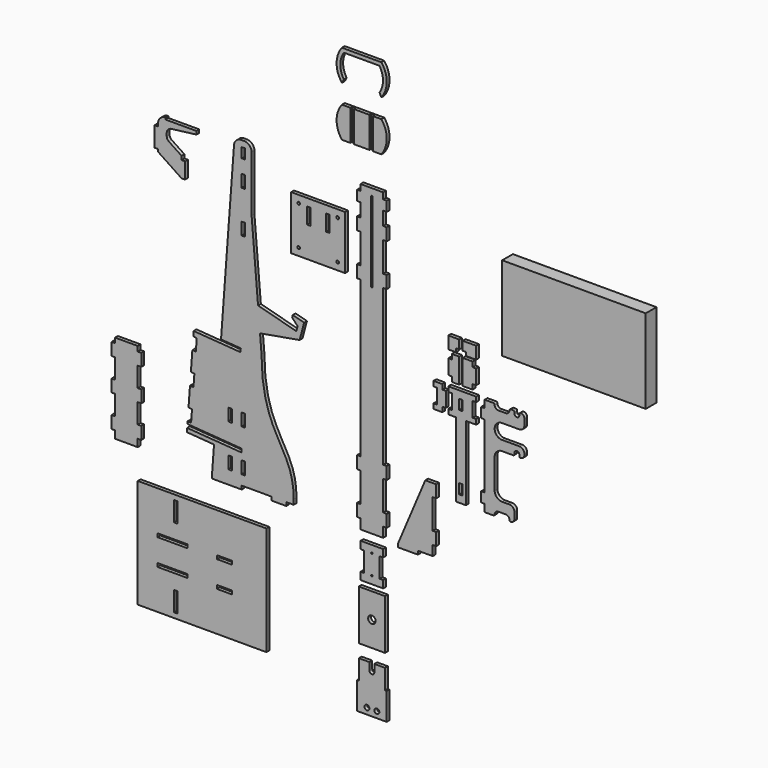
from build123d import *

# Parameters (mm, degrees)
F1_W     = 18.034
F1_H     = 63.5
F1_W_2   = 101.6
F1_H_2   = 18.034
F2_DEPTH = 18.034
F1_H_3   = 50.8
F1_W_3   = 152.4
F1_W_4   = 76.2
F1_W_5   = 276.2
F1_H_4   = 276.2
F1_R     = 6.985
F1_H_5   = 82.55
F1_R_2   = 12.7
F1_W_6   = 8.8265
F1_H_6   = 139.7
F1_W_7   = 9.2075
F1_H_7   = 101.6
F1_W_8   = 79.883
F1_H_8   = 158.75
F1_R_3   = 3.81
F1_W_9   = 134.366
F1_H_9   = 256.286
F1_R_4   = 19.05
F3_DEPTH = 9.017
F1_W_10  = 736.6
F1_H_10  = 431.8
F4_DEPTH = 68.58
F6_DEPTH = 18.034
F5_W     = 18.034
F5_H     = 50.8
F5_H_2   = 25.4
F5_H_3   = 76.2


# Not quite as in the source:
# - a variable given as a bare number and used for a length is read in inches; the dataset says mm whatever the document's units were


with BuildPart() as f2:
    # F1 (on Front) → F2 (new body)
    with BuildSketch(Plane.XZ):
        Polygon((312.166, -462.8884474277), (312.166, -399.3884474277), (274.066, -399.3884474277), (134.366, -729.5884474277), (235.966, -729.5884474277), (312.166, -729.5884474277), (312.166, -678.7884474277), (312.166, -615.2884474277), align=None)
        with Locations((321.183, -431.1384474277)):
            Rectangle(F1_W, F1_H)
        with Locations((321.183, -647.0384474277)):
            Rectangle(F1_W, F1_H)
        with Locations((185.166, -738.6054474277)):
            Rectangle(F1_W_2, F1_H_2)
    extrude(amount=F2_DEPTH)


with BuildPart() as f2b:
    # F1 (on Front) → F2, piece 2 (new body)
    with BuildSketch(Plane.XZ):
        with Locations((-1326.515, -329.5384474277)):
            Rectangle(F1_W, F1_H)
        with Locations((-1326.515, -494.6384474277)):
            Rectangle(F1_W, F1_H)
        with Locations((-1192.149, -494.6384474277)):
            Rectangle(F1_W, F1_H)
        with Locations((-1192.149, -329.5384474277)):
            Rectangle(F1_W, F1_H)
        Polygon((-1317.498, -729.5884474277), (-1201.166, -729.5884474277), (-1201.166, -691.4884474277), (-1201.166, -627.9884474277), (-1201.166, -526.3884474277), (-1201.166, -462.8884474277), (-1201.166, -361.2884474277), (-1201.166, -297.7884474277), (-1201.166, -272.3884474277), (-1317.498, -272.3884474277), (-1317.498, -297.7884474277), (-1317.498, -361.2884474277), (-1317.498, -462.8884474277), (-1317.498, -526.3884474277), (-1317.498, -627.9884474277), (-1317.498, -691.4884474277), align=None)
        with Locations((-1326.515, -659.7384474277)):
            Rectangle(F1_W, F1_H)
        with Locations((-1192.149, -659.7384474277)):
            Rectangle(F1_W, F1_H)
    extrude(amount=F2_DEPTH)


with BuildPart() as f2c:
    # F1 (on Front) → F2, piece 3 (new body)
    with BuildSketch(Plane.XZ):
        with BuildLine():
            Line((-707.3307957356, 795.6225112467), (-712.216, 729.5884474277))
            Line((-712.216, 729.5884474277), (-773.8601407698, -103.6649653974))
            Line((-773.8601407698, -103.6649653974), (-672.5370356253, -111.1608551959))
            Line((-672.5370356253, -111.1608551959), (-673.8675560645, -129.1457063591))
            Line((-673.8675560645, -129.1457063591), (-775.190661209, -121.6498165606))
            Line((-775.190661209, -121.6498165606), (-807.0481928526, -552.2730134248))
            Line((-807.0481928526, -552.2730134248), (-667.766, -562.5771189596))
            Line((-667.766, -562.5771189596), (-667.766, -580.6604021099))
            Line((-667.766, -580.6604021099), (-808.3787132919, -570.257864588))
            Line((-808.3787132919, -570.257864588), (-809.8591515271, -590.269177854))
            Line((-809.8591515271, -590.269177854), (-820.166, -729.5884474277))
            Line((-820.166, -729.5884474277), (-667.766, -729.5884474277))
            Line((-667.766, -729.5884474277), (-515.366, -729.5884474277))
            Line((-515.366, -729.5884474277), (-439.166, -729.5884474277))
            Line((-439.166, -729.5884474277), (-401.066, -729.5884474277))
            Line((-401.066, -729.5884474277), (-401.066, -704.1884474277))
            add(Edge.make_bspline(
                [(-566.166, -102.5384474277), (-566.166, -468.3954715729), (-401.066, -468.3954715729), (-401.066, -704.1884474277)],
                knots=[0, 0, 0, 0, 623.8916031652, 623.8916031652, 623.8916031652, 623.8916031652], degree=3))
            Line((-566.166, -102.5384474277), (-573.766897729, -11.3276746799))
            Line((-573.766897729, -11.3276746799), (-583.9832928314, 111.2690665494))
            Line((-583.9832928314, 111.2690665494), (-616.966, 507.0615525723))
            Line((-616.966, 507.0615525723), (-616.966, 544.2178131268))
            Line((-616.966, 544.2178131268), (-616.966, 627.7115525723))
            Line((-616.966, 627.7115525723), (-616.966, 659.4615525723))
            Line((-616.966, 659.4615525723), (-616.966, 761.0615525723))
            Line((-616.966, 761.0615525723), (-616.966, 792.8115525723))
            ThreePointArc((-616.966, 792.8115525723), (-628.1252316368, 819.7523209355), (-655.066, 830.9115525723))
            Line((-655.066, 830.9115525723), (-669.3346313064, 830.9115525723))
            ThreePointArc((-669.3346313064, 830.9115525723), (-695.2625359123, 820.7284607597), (-707.3307957356, 795.6225112467))
        make_face()
        with Locations((-727.583, -647.0384474277)):
            Rectangle(F1_W, F1_H, mode=Mode.SUBTRACT)
        with Locations((-658.749, -647.0384474277)):
            Rectangle(F1_W, F1_H, mode=Mode.SUBTRACT)
        with Locations((-727.583, -431.1384474277)):
            Rectangle(F1_W, F1_H, mode=Mode.SUBTRACT)
        with Locations((-658.749, -431.1384474277)):
            Rectangle(F1_W, F1_H, mode=Mode.SUBTRACT)
        with Locations((-658.749, 431.1384474277)):
            Rectangle(F1_W, F1_H, mode=Mode.SUBTRACT)
        with Locations((-658.749, 647.0384474277)):
            Rectangle(F1_W, F1_H, mode=Mode.SUBTRACT)
        with Locations((-658.749, 773.7615525723)):
            Rectangle(F1_W, F1_H_3, mode=Mode.SUBTRACT)
        Polygon((-387.7071649295, 58.6770365845), (-583.9832928314, 111.2690665494), (-573.766897729, -11.3276746799), (-370.5684031555, 24.5017023527), (-347.5593900459, 110.3725083098), (-405.8288655168, 125.9857672056), (-409.1158673896, 113.7185092117), (-381.1331611839, 83.2115525723), align=None)
        Polygon((-807.0481928526, -552.2730134248), (-775.190661209, -121.6498165606), (-914.5099307827, -111.3429680876), (-916.3839032324, -136.6737443738), (-898.3990520692, -138.004264813), (-903.0839831933, -201.3312055283), (-921.0688343564, -200.0006850891), (-928.5647241549, -301.3237902336), (-910.5798729918, -302.6543106729), (-915.2648041158, -365.9812513882), (-933.249655279, -364.650730949), (-940.7455450775, -465.9738360935), (-922.7606939143, -467.3043565327), (-927.4456250384, -530.631297248), (-945.4304762015, -529.3007768088), (-946.3674624264, -541.9661649519), align=None)
        Polygon((-809.8591515271, -590.269177854), (-808.3787132919, -570.257864588), (-947.6979828656, -559.951016115), (-949.1784211008, -579.9623293811), align=None)
        with Locations((-743.966, -738.6054474277)):
            Rectangle(F1_W_3, F1_H_2)
        with Locations((-477.266, -738.6054474277)):
            Rectangle(F1_W_4, F1_H_2)
    extrude(amount=F2_DEPTH)


with BuildPart() as f2d:
    # F1 (on Front) → F2, piece 4 (new body)
    with BuildSketch(Plane.XZ):
        with Locations((67.183, 647.0384474277)):
            Rectangle(F1_W, F1_H)
        with Locations((67.183, 431.1384474277)):
            Rectangle(F1_W, F1_H)
        with Locations((-67.183, 431.1384474277)):
            Rectangle(F1_W, F1_H)
        with Locations((-67.183, 647.0384474277)):
            Rectangle(F1_W, F1_H)
        with Locations((-67.183, -431.1384474277)):
            Rectangle(F1_W, F1_H)
        with Locations((-67.183, -647.0384474277)):
            Rectangle(F1_W, F1_H)
        with Locations((67.183, -647.0384474277)):
            Rectangle(F1_W, F1_H)
        with Locations((67.183, -431.1384474277)):
            Rectangle(F1_W, F1_H)
        Polygon((-58.166, -678.7884474277), (-58.166, -729.5884474277), (58.166, -729.5884474277), (58.166, -678.7884474277), (58.166, -615.2884474277), (58.166, -462.8884474277), (58.166, -399.3884474277), (58.166, 399.3884474277), (58.166, 462.8884474277), (58.166, 615.2884474277), (58.166, 678.7884474277), (58.166, 729.5884474277), (58.166, 748.3615525723), (58.166, 799.1615525723), (58.166, 830.9115525723), (-58.166, 830.9115525723), (-58.166, 799.1615525723), (-58.166, 748.3615525723), (-58.166, 729.5884474277), (-58.166, 678.7884474277), (-58.166, 615.2884474277), (-58.166, 462.8884474277), (-58.166, 399.3884474277), (-58.166, -399.3884474277), (-58.166, -462.8884474277), (-58.166, -615.2884474277), align=None)
        with BuildLine():
            Line((-3.81, 386.4115525723), (-3.81, 792.8115525723))
            ThreePointArc((-3.81, 792.8115525723), (0, 796.6215525723), (3.81, 792.8115525723))
            Line((3.81, 792.8115525723), (3.81, 386.4115525723))
            ThreePointArc((3.81, 386.4115525723), (0, 382.6015525723), (-3.81, 386.4115525723))
        make_face(mode=Mode.SUBTRACT)
        with Locations((-67.183, 773.7615525723)):
            Rectangle(F1_W, F1_H_3)
        with Locations((67.183, 773.7615525723)):
            Rectangle(F1_W, F1_H_3)
    extrude(amount=F2_DEPTH)


with BuildPart() as f2e:
    # F1 (on Front) → F2, piece 5 (new body)
    with BuildSketch(Plane.XZ):
        with Locations((-275.666, 540.4115525723)):
            Rectangle(F1_W_5, F1_H_4)
        with Locations((-375.666, 440.4115525723)):
            Circle(F1_R, mode=Mode.SUBTRACT)
        with Locations((-324.6245, 599.1365525723)):
            Rectangle(F1_W, F1_H_5, mode=Mode.SUBTRACT)
        with Locations((-375.666, 640.4115525723)):
            Circle(F1_R, mode=Mode.SUBTRACT)
        with Locations((-175.666, 440.4115525723)):
            Circle(F1_R, mode=Mode.SUBTRACT)
        with Locations((-226.7075, 599.1365525723)):
            Rectangle(F1_W, F1_H_5, mode=Mode.SUBTRACT)
        with Locations((-175.666, 640.4115525723)):
            Circle(F1_R, mode=Mode.SUBTRACT)
    extrude(amount=F2_DEPTH)


with BuildPart() as f2f:
    # F1 (on Front) → F2, piece 6 (new body)
    with BuildSketch(Plane.XZ):
        with BuildLine():
            ThreePointArc((-143.8170263099, 1275.6884474277), (-161.925, 1336.0134474277), (-143.8170263099, 1396.3384474277))
            Line((-143.8170263099, 1396.3384474277), (39.0420263099, 1396.3384474277))
            ThreePointArc((39.0420263099, 1396.3384474277), (57.15, 1336.0134474277), (39.0420263099, 1275.6884474277))
            Line((39.0420263099, 1275.6884474277), (48.7774866864, 1256.6384474277))
            ThreePointArc((48.7774866864, 1256.6384474277), (76.2, 1336.0134474277), (48.7774866864, 1415.3884474277))
            Line((48.7774866864, 1415.3884474277), (-153.5524866864, 1415.3884474277))
            ThreePointArc((-153.5524866864, 1415.3884474277), (-180.975, 1336.0134474277), (-153.5524866864, 1256.6384474277))
            Line((-153.5524866864, 1256.6384474277), (-143.8170263099, 1275.6884474277))
        make_face()
    extrude(amount=F2_DEPTH)


with BuildPart() as f2g:
    # F1 (on Front) → F2, piece 7 (new body)
    with BuildSketch(Plane.XZ):
        with BuildLine():
            Line((-12.5095, -1313.7884474277), (-66.9925, -1313.7884474277))
            Line((-66.9925, -1313.7884474277), (-66.9925, -1415.3884474277))
            Line((-66.9925, -1415.3884474277), (-66.9925, -1555.0884474277))
            Line((-66.9925, -1555.0884474277), (67.3735, -1555.0884474277))
            Line((67.3735, -1555.0884474277), (67.3735, -1415.3884474277))
            Line((67.3735, -1415.3884474277), (67.3735, -1313.7884474277))
            Line((67.3735, -1313.7884474277), (12.8905, -1313.7884474277))
            Line((12.8905, -1313.7884474277), (12.8905, -1351.8884474277))
            ThreePointArc((12.8905, -1351.8884474277), (0.1905, -1364.5884474277), (-12.5095, -1351.8884474277))
            Line((-12.5095, -1351.8884474277), (-12.5095, -1313.7884474277))
        make_face()
        with Locations((-25.2095, -1523.3384474277)):
            Circle(F1_R_2, mode=Mode.SUBTRACT)
        with Locations((25.5905, -1523.3384474277)):
            Circle(F1_R_2, mode=Mode.SUBTRACT)
        with Locations((71.78675, -1485.2384474277)):
            Rectangle(F1_W_6, F1_H_6)
        with Locations((-71.59625, -1485.2384474277)):
            Rectangle(F1_W_7, F1_H_6)
    extrude(amount=F2_DEPTH)


with BuildPart() as f2h:
    # F1 (on Front) → F2, piece 8 (new body)
    with BuildSketch(Plane.XZ):
        with BuildLine():
            Line((-976.2594103813, 640.4115525723), (-976.2594103813, 659.4615525723))
            Line((-976.2594103813, 659.4615525723), (-1041.1487953654, 702.7211425617))
            ThreePointArc((-1041.1487953654, 702.7211425617), (-1049.45394519, 711.8700287293), (-1052.4594103813, 723.8552200379))
            Line((-1052.4594103813, 723.8552200379), (-1052.4594103813, 738.6388842214))
            ThreePointArc((-1052.4594103813, 738.6388842214), (-1046.101236047, 755.4486693276), (-1030.2098926399, 763.8427422899))
            Line((-1030.2098926399, 763.8427422899), (-900.0594103813, 780.1115525723))
            Line((-900.0594103813, 780.1115525723), (-900.0594103813, 796.4945525723))
            Line((-900.0594103813, 796.4945525723), (-1058.8094103813, 796.4945525723))
            Line((-1058.8094103813, 796.4945525723), (-1058.8094103813, 805.5115525723))
            ThreePointArc((-1058.8094103813, 805.5115525723), (-1085.7501787445, 794.3523209355), (-1096.9094103813, 767.4115525723))
            Line((-1096.9094103813, 767.4115525723), (-1096.9094103813, 752.5948859056))
            Line((-1096.9094103813, 752.5948859056), (-1096.9094103813, 650.9948859056))
            Line((-1096.9094103813, 650.9948859056), (-1096.9094103813, 638.2948859056))
            Line((-1096.9094103813, 638.2948859056), (-976.2594103813, 557.8615525723))
            Line((-976.2594103813, 557.8615525723), (-958.2254103813, 557.8615525723))
            Line((-958.2254103813, 557.8615525723), (-958.2254103813, 640.4115525723))
            Line((-958.2254103813, 640.4115525723), (-976.2594103813, 640.4115525723))
        make_face()
        with Locations((-1105.9264103813, 701.7948859056)):
            Rectangle(F1_W, F1_H_7)
    extrude(amount=F2_DEPTH)


with BuildPart() as f2i:
    # F1 (on Front) → F2, piece 9 (new body)
    with BuildSketch(Plane.XZ):
        with BuildLine():
            ThreePointArc((48.7774866864, 999.4634474277), (69.1511726145, 1036.8492081472), (76.2, 1078.8384474277))
            ThreePointArc((76.2, 1078.8384474277), (69.1511726145, 1120.8276867083), (48.7774866864, 1158.2134474277))
            Line((48.7774866864, 1158.2134474277), (5.588, 1158.2134474277))
            Line((5.588, 1158.2134474277), (5.588, 999.4634474277))
            Line((5.588, 999.4634474277), (48.7774866864, 999.4634474277))
        make_face()
    extrude(amount=F2_DEPTH)



with BuildPart() as f2j:
    # F1 (on Front) → F2, piece 10 (new body)
    with BuildSketch(Plane.XZ):
        with Locations((-52.3875, 1078.8384474277)):
            Rectangle(F1_W_8, F1_H_8)
    extrude(amount=F2_DEPTH)


with BuildPart() as f2k:
    # F1 (on Front) → F2, piece 11 (new body)
    with BuildSketch(Plane.XZ):
        with BuildLine():
            ThreePointArc((-153.5524866864, 1158.2134474277), (-173.9261725074, 1120.8276870182), (-180.975, 1078.8384480836))
            ThreePointArc((-180.975, 1078.8384480836), (-173.9261727216, 1036.8492084571), (-153.5524866864, 999.4634474277))
            Line((-153.5524866864, 999.4634474277), (-110.363, 999.4634474277))
            Line((-110.363, 999.4634474277), (-110.363, 1158.2134474277))
            Line((-110.363, 1158.2134474277), (-153.5524866864, 1158.2134474277))
        make_face()
    extrude(amount=F2_DEPTH)


with BuildPart() as f2l:
    # F1 (on Front) → F2, piece 12 (new body)
    with BuildSketch(Plane.XZ):
        Polygon((58.166, -780.3884474277), (-57.785, -780.3884474277), (-57.785, -818.4884474277), (-39.751, -818.4884474277), (-39.751, -920.0884474277), (-57.785, -920.0884474277), (-57.785, -958.1884474277), (58.166, -958.1884474277), (58.166, -920.0884474277), (40.132, -920.0884474277), (40.132, -818.4884474277), (58.166, -818.4884474277), align=None)
        with Locations((0.1905, -920.0884474277)):
            Circle(F1_R_3, mode=Mode.SUBTRACT)
        with Locations((0.1905, -818.4884474277)):
            Circle(F1_R_3, mode=Mode.SUBTRACT)
    extrude(amount=F2_DEPTH)


with BuildPart() as f2m:
    # F1 (on Front) → F2, piece 13 (new body)
    with BuildSketch(Plane.XZ):
        with Locations((0.1905, -1118.0814474277)):
            Rectangle(F1_W_9, F1_H_9)
        with Locations((0, -1118.0814474277)):
            Circle(F1_R_4, mode=Mode.SUBTRACT)
    extrude(amount=F2_DEPTH)


with BuildPart() as f2n:
    # F1 (on Front) → F2, piece 14 (new body)
    with BuildSketch(Plane.XZ):
        Polygon((-540.766, -881.9884474277), (-1201.166, -881.9884474277), (-1201.166, -1440.7884474277), (-540.766, -1440.7884474277), (-540.766, -1161.3884474277), (-540.766, -994.3783283234), align=None)
        with Locations((-1006.983, -1364.5884474277)):
            Rectangle(F1_W, F1_H_7, mode=Mode.SUBTRACT)
        with Locations((-1023.366, -1228.5714474277)):
            Rectangle(F1_W_3, F1_H_2, mode=Mode.SUBTRACT)
        with Locations((-756.666, -1228.5714474277)):
            Rectangle(F1_W_4, F1_H_2, mode=Mode.SUBTRACT)
        with Locations((-1023.366, -1094.2054474277)):
            Rectangle(F1_W_3, F1_H_2, mode=Mode.SUBTRACT)
        with Locations((-1006.983, -958.1884474277)):
            Rectangle(F1_W, F1_H_7, mode=Mode.SUBTRACT)
        with Locations((-756.666, -1094.2054474277)):
            Rectangle(F1_W_4, F1_H_2, mode=Mode.SUBTRACT)
    extrude(amount=F2_DEPTH)


with BuildPart() as f2i_1:
    add(f2i.part)

    add(f2j.part)  # F3 merges F2j

    add(f2k.part)  # F3 merges F2k
    # F1 (on Front) → F3 (join)
    with BuildSketch(Plane.XZ):
        with Locations((-101.346, 1078.8384474277)):
            Rectangle(F1_W, F1_H_8)
        with Locations((-3.429, 1078.8384474277)):
            Rectangle(F1_W, F1_H_8)
    extrude(amount=F3_DEPTH)


with BuildPart() as f4:
    # F1 (on Front) → F4 (new body)
    with BuildSketch(Plane.XZ):
        with Locations((1077.2890025383, 540.4115525723)):
            Rectangle(F1_W_10, F1_H_10)
    extrude(amount=F4_DEPTH)


with BuildPart() as f6:
    # F5 (on Front) → F6 (new body)
    with BuildSketch(Plane.XZ):
        Polygon((410.083, 114.3), (410.083, 88.9), (448.183, 88.9), (448.183, 215.9), (410.083, 215.9), (410.083, 190.5), (392.049, 190.5), (392.049, 114.3), align=None)
    extrude(amount=F6_DEPTH)


with BuildPart() as f6b:
    # F5 (on Front) → F6, piece 2 (new body)
    with BuildSketch(Plane.XZ):
        Polygon((466.217, 215.9), (466.217, 88.9), (517.017, 88.9), (517.017, 114.3), (535.051, 114.3), (535.051, 190.5), (517.017, 190.5), (517.017, 215.9), align=None)
    extrude(amount=F6_DEPTH)


with BuildPart() as f6c:
    # F5 (on Front) → F6, piece 3 (new body)
    with BuildSketch(Plane.XZ):
        Polygon((504.317, 63.5), (410.083, 63.5), (410.083, 38.1), (410.083, -38.1), (410.083, -63.5), (431.8, -63.5), (431.8, -444.5), (482.6, -444.5), (482.6, -63.5), (504.317, -63.5), (517.017, -63.5), (517.017, -38.1), (517.017, 38.1), (517.017, 63.5), align=None)
        with Locations((457.2, -381)):
            Rectangle(F5_W, F5_H, mode=Mode.SUBTRACT)
        with Locations((457.2, 0)):
            Rectangle(F5_W, F5_H, mode=Mode.SUBTRACT)
        with Locations((401.066, 50.8)):
            Rectangle(F5_W, F5_H_2)
        with Locations((401.066, -50.8)):
            Rectangle(F5_W, F5_H_2)
        with Locations((526.034, -50.8)):
            Rectangle(F5_W, F5_H_2)
        with Locations((526.034, 50.8)):
            Rectangle(F5_W, F5_H_2)
    extrude(amount=F6_DEPTH)


with BuildPart() as f6d:
    # F5 (on Front) → F6, piece 4 (new body)
    with BuildSketch(Plane.XZ):
        Polygon((361.315, -38.1), (361.315, 38.1), (361.315, 63.5), (334.3275, 63.5), (334.3275, 38.1), (334.3275, -38.1), (334.3275, -63.5), (361.315, -63.5), align=None)
        with Locations((325.3105, 50.8)):
            Rectangle(F5_W, F5_H_2)
        with Locations((325.3105, -50.8)):
            Rectangle(F5_W, F5_H_2)
        with Locations((370.332, 0)):
            Rectangle(F5_W, F5_H_3)
    extrude(amount=F6_DEPTH)


with BuildPart() as f6e:
    # F5 (on Front) → F6, piece 5 (new body)
    with BuildSketch(Plane.XZ):
        with BuildLine():
            Line((578.485, 25.4), (560.451, 25.4))
            Line((560.451, 25.4), (560.451, -25.4))
            Line((560.451, -25.4), (578.485, -25.4))
            Line((578.485, -25.4), (578.485, -355.6))
            Line((578.485, -355.6), (560.451, -355.6))
            Line((560.451, -355.6), (560.451, -406.4))
            Line((560.451, -406.4), (578.485, -406.4))
            Line((578.485, -406.4), (578.485, -444.5))
            Line((578.485, -444.5), (623.5065, -444.5))
            ThreePointArc((623.5065, -444.5), (627.9966280605, -442.6401280605), (629.8565, -438.15))
            ThreePointArc((629.8565, -438.15), (635.4361158184, -424.6796158184), (648.9065, -419.1))
            Line((648.9065, -419.1), (687.0065, -419.1))
            ThreePointArc((687.0065, -419.1), (700.4768841816, -424.6796158184), (706.0565, -438.15))
            ThreePointArc((706.0565, -438.15), (707.9163719395, -442.6401280605), (712.4065, -444.5))
            ThreePointArc((712.4065, -444.5), (725.8768841816, -438.9203841816), (731.4565, -425.45))
            Line((731.4565, -425.45), (731.4565, -393.7))
            ThreePointArc((731.4565, -393.7), (724.0170122421, -375.7394877579), (706.0565, -368.3))
            Line((706.0565, -368.3), (667.9565, -368.3))
            ThreePointArc((667.9565, -368.3), (641.0157316368, -357.1407683632), (629.8565, -330.2))
            Line((629.8565, -330.2), (629.8565, -177.8))
            ThreePointArc((629.8565, -177.8), (641.0157316368, -150.8592316368), (667.9565, -139.7))
            Line((667.9565, -139.7), (725.1065, -139.7))
            ThreePointArc((725.1065, -139.7), (729.5966280605, -137.8401280605), (731.4565, -133.35))
            Line((731.4565, -133.35), (731.4565, -127))
            ThreePointArc((731.4565, -127), (735.1762438789, -118.0197438789), (744.1565, -114.3))
            ThreePointArc((744.1565, -114.3), (753.1367561211, -118.0197438789), (756.8565, -127))
            Line((756.8565, -127), (756.8565, -133.35))
            ThreePointArc((756.8565, -133.35), (758.7163719395, -137.8401280605), (763.2065, -139.7))
            ThreePointArc((763.2065, -139.7), (776.6768841816, -134.1203841816), (782.2565, -120.65))
            Line((782.2565, -120.65), (782.2565, -114.3))
            ThreePointArc((782.2565, -114.3), (774.8170122421, -96.3394877579), (756.8565, -88.9))
            Line((756.8565, -88.9), (667.9565, -88.9))
            ThreePointArc((667.9565, -88.9), (641.0157316368, -77.7407683632), (629.8565, -50.8))
            ThreePointArc((629.8565, -50.8), (641.0157316368, -23.8592316368), (667.9565, -12.7))
            Line((667.9565, -12.7), (756.8565, -12.7))
            ThreePointArc((756.8565, -12.7), (774.8170122421, -5.2605122421), (782.2565, 12.7))
            Line((782.2565, 12.7), (782.2565, 44.45))
            ThreePointArc((782.2565, 44.45), (776.6768841816, 57.9203841816), (763.2065, 63.5))
            ThreePointArc((763.2065, 63.5), (758.7163719395, 61.6401280605), (756.8565, 57.15))
            Line((756.8565, 57.15), (756.8565, 50.8))
            ThreePointArc((756.8565, 50.8), (753.1367561211, 41.8197438789), (744.1565, 38.1))
            ThreePointArc((744.1565, 38.1), (735.1762438789, 41.8197438789), (731.4565, 50.8))
            Line((731.4565, 50.8), (731.4565, 57.15))
            ThreePointArc((731.4565, 57.15), (729.5966280605, 61.6401280605), (725.1065, 63.5))
            Line((725.1065, 63.5), (712.4065, 63.5))
            ThreePointArc((712.4065, 63.5), (707.9163719395, 61.6401280605), (706.0565, 57.15))
            ThreePointArc((706.0565, 57.15), (700.4768841816, 43.6796158184), (687.0065, 38.1))
            Line((687.0065, 38.1), (648.9065, 38.1))
            ThreePointArc((648.9065, 38.1), (635.4361158184, 43.6796158184), (629.8565, 57.15))
            ThreePointArc((629.8565, 57.15), (627.9966280605, 61.6401280605), (623.5065, 63.5))
            Line((623.5065, 63.5), (578.485, 63.5))
            Line((578.485, 63.5), (578.485, 25.4))
        make_face()
    extrude(amount=F6_DEPTH)


with BuildPart() as f6f:
    # F5 (on Front) → F6, piece 6 (new body)
    with BuildSketch(Plane.XZ):
        Polygon((431.8, 248.1941320505), (448.183, 248.1941320505), (448.183, 293.2156320505), (392.049, 293.2156320505), (392.049, 230.1601320505), (431.8, 230.1601320505), align=None)
    extrude(amount=F6_DEPTH)


with BuildPart() as f6g:
    # F5 (on Front) → F6, piece 7 (new body)
    with BuildSketch(Plane.XZ):
        Polygon((535.051, 293.2156320505), (466.217, 293.2156320505), (466.217, 248.1941320505), (482.6, 248.1941320505), (482.6, 230.1601320505), (535.051, 230.1601320505), align=None)
    extrude(amount=F6_DEPTH)


solid = Compound([f2.part, f2b.part, f2c.part, f2d.part, f2e.part, f2f.part, f2g.part, f2h.part, f2l.part, f2m.part, f2n.part, f2i_1.part, f4.part, f6.part, f6b.part, f6c.part, f6d.part, f6e.part, f6f.part, f6g.part])
